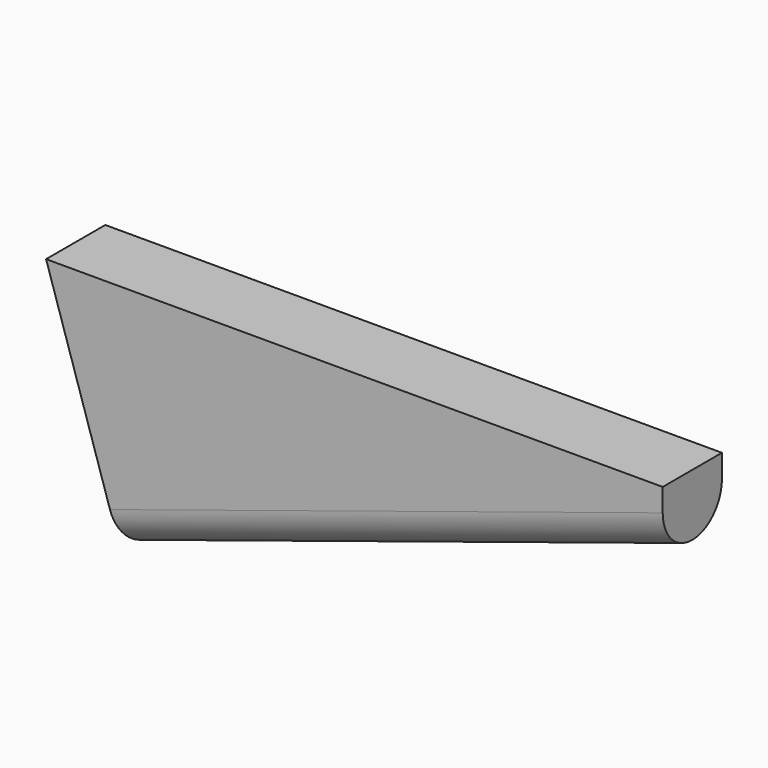
from build123d import *

# Parameters (mm, degrees)
F1_DEPTH = 3
F2_R     = 2.99999


# Not quite as in the source:
# - a fillet or chamfer is up to 0.001 mm smaller than in the source, because OpenCascade refuses the exact size


with BuildPart() as f1:
    # F0 (on Front) → F1 (new body, symmetric)
    with BuildSketch(Plane.XZ):
        Polygon((50, 0), (0, 0), (6.0951397114, -19.0486028857), (50, -5), align=None)
    extrude(amount=F1_DEPTH, both=True)

    # F2 (radius 3 in the source; OpenCascade refuses exactly that, so slightly less here)
    f2_edges = [f1.edges().sort_by_distance(p)[0] for p in [
        (28.04757, -3, -12.024301),
        (28.04757, 3, -12.024301),
    ]]
    fillet(f2_edges, radius=F2_R)


solid = f1.part
